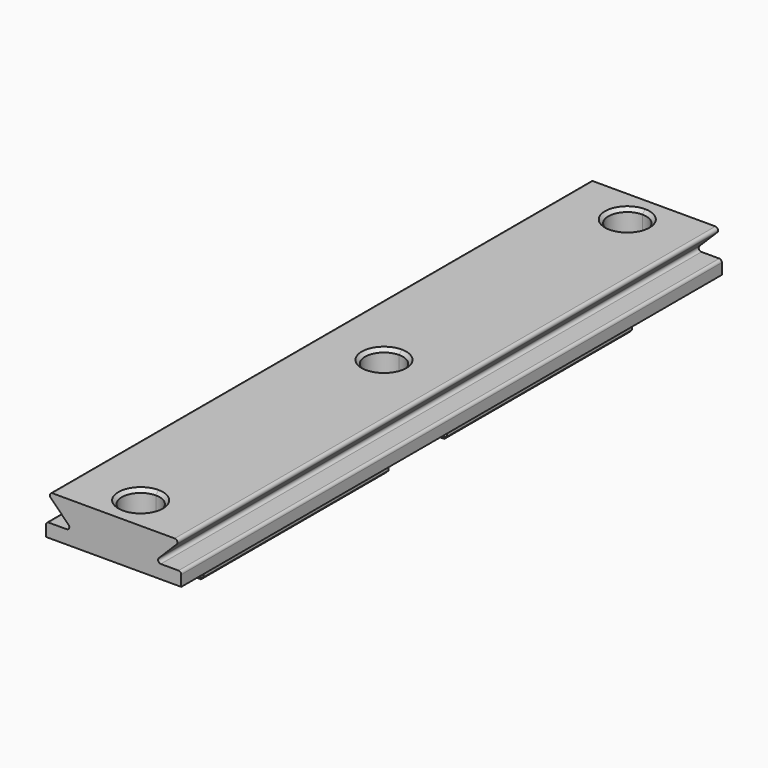
from build123d import *

# Parameters (mm, degrees)
F1_DEPTH  = 100
F2_W      = 5
F2_H      = 10
F3_DEPTH  = 5
F4_R      = 0.875
F5_DEPTH  = 25
F6_R      = 0.4
F8_DEPTH  = 3.5
F9_DEPTH  = 11.001
F10_SIZE  = 0.5
F11_W     = 10
F11_H     = 5
F12_DEPTH = 25
F13_SIZE  = 0.4


with BuildPart() as f1:
    # F0 (on Front) → F1 (new body)
    with BuildSketch(Plane.XZ):
        Polygon((2.5, -2.5), (5, -2.5), (5, 2.5), (10, 2.5), (10, 4.5), (6, 4.5), (10, 8.5), (6, 8.5), (-6, 8.5), (-10, 8.5), (-6, 4.5), (-10, 4.5), (-10, 2.5), (-5, 2.5), (-5, -2.5), (-2.5, -2.5), (-2.5, 2.5), (2.5, 2.5), align=None)
    extrude(amount=F1_DEPTH)

    # F2 (on face) → F3 (join)
    with BuildSketch(Plane(origin=(0, 0, 2.5), x_dir=(1, 0, 0), z_dir=(0, 0, -1))):
        with Locations((0, 95)):
            Rectangle(F2_W, F2_H)
        Polygon((-2.5, 50), (-2.5, 45), (2.5, 45), (2.5, 50), (2.5, 55), (-2.5, 55), align=None)
        with Locations((0, 5)):
            Rectangle(F2_W, F2_H)
    extrude(amount=F3_DEPTH)

    # F4 (on face) → F5 (cut)
    with BuildSketch(Plane.YZ.offset(5)):
        with Locations((-85, 0)):
            Circle(F4_R)
        with Locations((-40, 0)):
            Circle(F4_R)
    extrude(amount=-F5_DEPTH, mode=Mode.SUBTRACT)

    # F6
    f6_edges = [f1.edges().sort_by_distance(p)[0] for p in [
        (10, -50, 4.5),
        (-10, -50, 4.5),
        (-6, -50, 4.5),
        (6, -50, 4.5),
        (10, -50, 8.5),
        (-10, -50, 8.5),
    ]]
    fillet(f6_edges, radius=F6_R)

    # F7 (on face) → F8 (cut)
    with BuildSketch(Plane.XY.offset(8.5)):
        with BuildLine():
            ThreePointArc((0, -92.2), (-2.8, -95), (0, -97.8))
            Line((0, -97.8), (0, -96.5))
            ThreePointArc((0, -96.5), (-1.5, -95), (0, -93.5))
            Line((0, -93.5), (0, -92.2))
        make_face()
        with BuildLine():
            ThreePointArc((0, -2.2), (-2.8, -5), (0, -7.8))
            Line((0, -7.8), (0, -6.5))
            ThreePointArc((0, -6.5), (-1.5, -5), (0, -3.5))
            Line((0, -3.5), (0, -2.2))
        make_face()
        with BuildLine():
            Line((0, -6.5), (0, -7.8))
            ThreePointArc((0, -7.8), (1.9798989873, -6.9798989873), (2.8, -5))
            ThreePointArc((2.8, -5), (1.9798989873, -3.0201010127), (0, -2.2))
            Line((0, -2.2), (0, -3.5))
            ThreePointArc((0, -3.5), (1.0606601718, -3.9393398282), (1.5, -5))
            ThreePointArc((1.5, -5), (1.0606601718, -6.0606601718), (0, -6.5))
        make_face()
        with BuildLine():
            ThreePointArc((0, -47.2), (-2.8, -50), (0, -52.8))
            Line((0, -52.8), (0, -51.5))
            ThreePointArc((0, -51.5), (-1.5, -50), (0, -48.5))
            Line((0, -48.5), (0, -47.2))
        make_face()
        with BuildLine():
            Line((0, -51.5), (0, -52.8))
            ThreePointArc((0, -52.8), (1.9798989873, -51.9798989873), (2.8, -50))
            ThreePointArc((2.8, -50), (1.9798989873, -48.0201010127), (0, -47.2))
            Line((0, -47.2), (0, -48.5))
            ThreePointArc((0, -48.5), (1.0606601718, -48.9393398282), (1.5, -50))
            ThreePointArc((1.5, -50), (1.0606601718, -51.0606601718), (0, -51.5))
        make_face()
        with BuildLine():
            Line((0, -96.5), (0, -97.8))
            ThreePointArc((0, -97.8), (1.9798989873, -96.9798989873), (2.8, -95))
            ThreePointArc((2.8, -95), (1.9798989873, -93.0201010127), (0, -92.2))
            Line((0, -92.2), (0, -93.5))
            ThreePointArc((0, -93.5), (1.0606601718, -93.9393398282), (1.5, -95))
            ThreePointArc((1.5, -95), (1.0606601718, -96.0606601718), (0, -96.5))
        make_face()
    extrude(amount=-F8_DEPTH, mode=Mode.SUBTRACT)

    # F9 (cut, through all): faces of the model
    f9_faces = [f1.faces().sort_by_distance(p)[0] for p in [
        (0, -5, 8.5),
        (0, -50, 8.5),
        (0, -95, 8.5),
    ]]
    extrude(f9_faces, amount=-F9_DEPTH, mode=Mode.SUBTRACT)

    # F10
    f10_edges = [f1.edges().sort_by_distance(p)[0] for p in [
        (0, -2.2, 8.5),
        (0, -47.2, 8.5),
        (0, -92.2, 8.5),
        (0, -6.5, 5),
        (0, -51.5, 5),
        (0, -96.5, 5),
        (0, -96.5, -2.5),
        (0, -51.5, -2.5),
        (0, -6.5, -2.5),
    ]]
    chamfer(f10_edges, length=F10_SIZE)

    # F11 (on face) → F12 (cut)
    with BuildSketch(Plane(origin=(-5, 0, 0), x_dir=(0, -1, 0), z_dir=(-1, 0, 0))):
        with Locations((5, 0)):
            Rectangle(F11_W, F11_H)
        with Locations((50, 0)):
            Rectangle(F11_W, F11_H)
        with Locations((95, 0)):
            Rectangle(F11_W, F11_H)
    extrude(amount=-F12_DEPTH, mode=Mode.SUBTRACT)

    # F13
    f13_edges = [f1.edges().sort_by_distance(p)[0] for p in [
        (5, -72.5, -2.5),
        (3.75, -90, -2.5),
        (2.5, -72.5, -2.5),
        (3.75, -55, -2.5),
        (-3.75, -55, -2.5),
        (-2.5, -72.5, -2.5),
        (-3.75, -90, -2.5),
        (-5, -72.5, -2.5),
        (-3.75, -10, -2.5),
        (-2.5, -27.5, -2.5),
        (-3.75, -45, -2.5),
        (-5, -27.5, -2.5),
        (5, -27.5, -2.5),
        (3.75, -45, -2.5),
        (2.5, -27.5, -2.5),
        (3.75, -10, -2.5),
        (2.5, -90, 0),
        (5, -90, 0),
        (3.75, -90, 2.5),
        (-5, -90, 0),
        (-2.5, -90, 0),
        (-3.75, -90, 2.5),
        (2.5, -45, 0),
        (5, -45, 0),
        (3.75, -45, 2.5),
        (-5, -45, 0),
        (-2.5, -45, 0),
        (-3.75, -45, 2.5),
        (2.5, -55, 0),
        (3.75, -55, 2.5),
        (5, -55, 0),
        (-5, -55, 0),
        (-3.75, -55, 2.5),
        (-2.5, -55, 0),
        (-5, -10, 0),
        (-3.75, -10, 2.5),
        (-2.5, -10, 0),
        (2.5, -10, 0),
        (3.75, -10, 2.5),
        (5, -10, 0),
        (5, -27.5, 2.5),
        (2.5, -27.5, 2.5),
        (-2.5, -27.5, 2.5),
        (-5, -27.5, 2.5),
        (5, -72.5, 2.5),
        (2.5, -72.5, 2.5),
        (-2.5, -72.5, 2.5),
        (-5, -72.5, 2.5),
    ]]
    chamfer(f13_edges, length=F13_SIZE)


solid = f1.part
